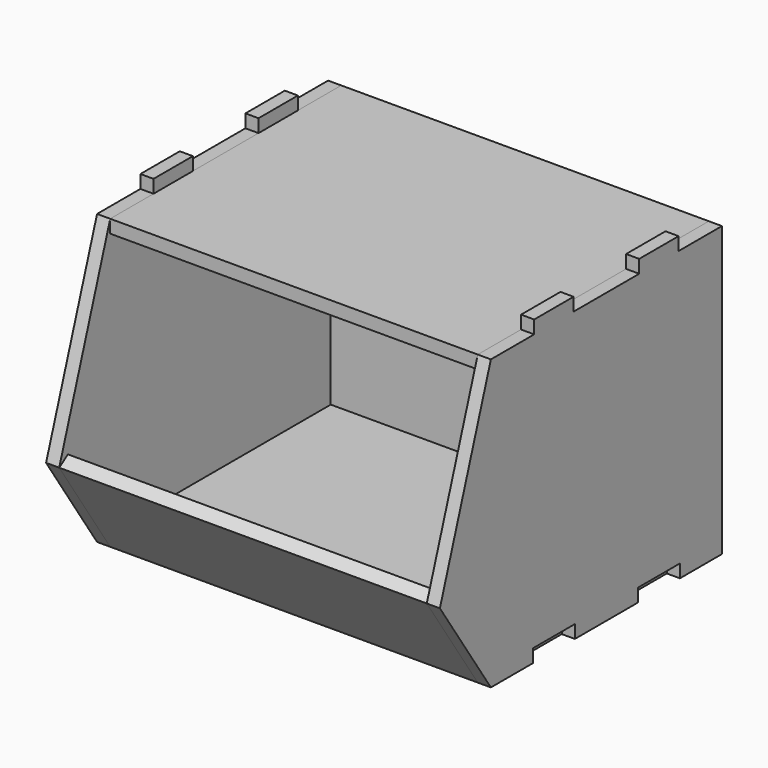
from build123d import *

# Parameters (mm, degrees)
F3_START  = 177.8
F3_DEPTH  = 12.7
F5_W      = 355.6
F5_H      = 279.4
F6_DEPTH  = 12.7
F7_W      = 355.6
F7_H      = 111.125
F8_DEPTH  = 12.7
F9_W      = 355.6
F9_H      = 268.8338474026
F10_DEPTH = 12.7
F11_W     = 355.6
F11_H     = 254
F12_DEPTH = 12.7


# Not quite as in the source:
# - a variable given as a bare number and used for a length is read in inches; the dataset says mm whatever the document's units were


with BuildPart() as f3:
    # F2 (on Right) → F3 (new body)
    with BuildSketch(Plane.YZ.offset(F3_START)):
        Polygon((139.7, -139.7), (139.7, 139.7), (87.3125, 139.7), (87.3125, 152.4), (39.6875, 152.4), (39.6875, 139.7), (0, 139.7), (-39.6875, 139.7), (-39.6875, 152.4), (-87.3125, 152.4), (-87.3125, 139.7), (-139.7, 139.7), (-201.3526883174, -47.2461647727), (-139.7, -139.7), (-88.9, -139.7), (-88.9, -127), (-38.1, -127), (-38.1, -139.7), (0, -139.7), (38.1, -139.7), (38.1, -127), (88.9, -127), (88.9, -139.7), align=None)
    extrude(amount=F3_DEPTH)


with BuildPart() as f4_1:
    # F4: instance of F3
    add(f3.part.mirror(Plane.YZ))


with BuildPart() as f6:
    # F5 (on face) → F6 (new body)
    with BuildSketch(Plane.XY.offset(139.7)):
        Rectangle(F5_W, F5_H)
    extrude(amount=-F6_DEPTH)


with BuildPart() as f8:
    # F7 (on face) → F8 (new body)
    with BuildSketch(Plane(origin=(0, -161.1828435034, -107.4845147117), x_dir=(1, 0, 0), z_dir=(0, -0.8319805195, -0.5548048443))):
        with Locations((0, 16.8410581705)):
            Rectangle(F7_W, F7_H)
    extrude(amount=-F8_DEPTH)


with BuildPart() as f10:
    # F9 (on face) → F10 (new body)
    with BuildSketch(Plane(origin=(0, 0, -139.7), x_dir=(1, 0, 0), z_dir=(0, 0, -1))):
        with Locations((0, -5.2830762987)):
            Rectangle(F9_W, F9_H)
    extrude(amount=-F10_DEPTH)


with BuildPart() as f12:
    # F11 (on face) → F12 (new body)
    with BuildSketch(Plane(origin=(0, 139.7, 0), x_dir=(-1, 0, 0), z_dir=(0, 1, 0))):
        Rectangle(F11_W, F11_H)
    extrude(amount=-F12_DEPTH)


solid = Compound([f3.part, f4_1.part, f6.part, f8.part, f10.part, f12.part])
